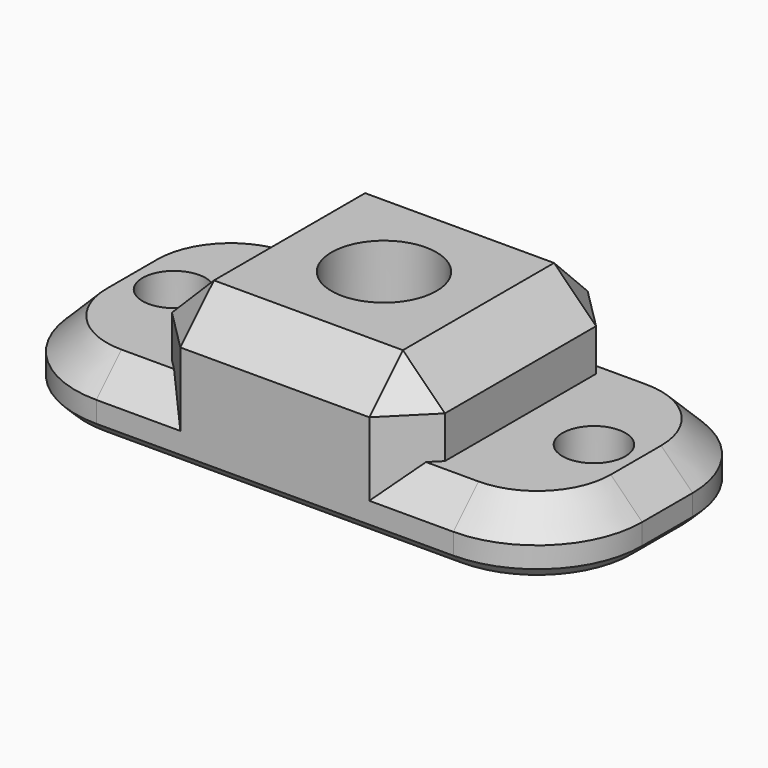
from build123d import *

# Parameters (mm, degrees)
F0_W         = 13
F0_H         = 13
F0_R         = 2.5
F1_DEPTH     = 7
F0_W_2       = 7
F0_R_2       = 1.5
F2_DEPTH     = 3
F3_SIZE      = 2
F4_R         = 5
F5_SIZE      = 1.5
F6_T1_DEPTH  = 3
F6_T3_DEPTH  = 17
F6_T6_ANGLE  = 90
F6_T8_ANGLE  = 90
F6_T10_ANGLE = 90
F6_T12_ANGLE = 90


# Not quite as in the source:
# - a fillet or chamfer that OpenCascade refuses, or shapes differently, is made with other operations: its cross-section is extruded or revolved along the edge and cut away or added


with BuildPart() as f1:
    # F0 (on Top) → F1 (new body)
    with BuildSketch(Plane.XY):
        Rectangle(F0_W, F0_H)
        Circle(F0_R, mode=Mode.SUBTRACT)
    extrude(amount=F1_DEPTH)

    # F0 (on Top) → F2 (join)
    with BuildSketch(Plane.XY):
        with Locations((-10, 0)):
            Rectangle(F0_W_2, F0_H)
        with Locations((-10, 0)):
            Circle(F0_R_2, mode=Mode.SUBTRACT)
        with Locations((10, 0)):
            Rectangle(F0_W_2, F0_H)
        with Locations((10, 0)):
            Circle(F0_R_2, mode=Mode.SUBTRACT)
    extrude(amount=F2_DEPTH)

    # F3
    f3_edges = [f1.edges().sort_by_distance(p)[0] for p in [
        (-2.5, 0, 0),
        (6.5, 0, 7),
        (-6.5, 0, 7),
        (0, -6.5, 7),
        (0, 6.5, 7),
        (-6.5, -6.5, 5),
        (6.5, -6.5, 5),
        (-6.5, 6.5, 5),
        (6.5, 6.5, 5),
    ]]
    chamfer(f3_edges, length=F3_SIZE)

    # F4
    f4_edges = [f1.edges().sort_by_distance(p)[0] for p in [
        (-13.5, 6.5, 1.5),
        (-13.5, -6.5, 1.5),
        (13.5, -6.5, 1.5),
        (13.5, 6.5, 1.5),
    ]]
    fillet(f4_edges, radius=F4_R)

    # F5
    f5_edges = [f1.edges().sort_by_distance(p)[0] for p in [
        (-12.035534, -5.035534, 3),
        (12.035534, -5.035534, 3),
        (7.5, 6.5, 3),
        (12.035534, 5.035534, 3),
        (13.5, 0, 3),
        (7.5, -6.5, 3),
        (-7.5, 6.5, 3),
        (-7.5, -6.5, 3),
        (-13.5, 0, 3),
        (-12.035534, 5.035534, 3),
    ]]
    chamfer(f5_edges, length=F5_SIZE)

    # F6: chamfer of 0.5 on 11 edges, made by hand

    # F6_s2 → F6_t1 (cut)
    with BuildSketch(Plane.XZ.offset(-1.5)):
        Polygon((-13, 0), (-13.5, 0.5), (-13.5, 0), align=None)
        Polygon((13.5, 0.5), (13, 0), (13.5, 0), align=None)
    extrude(amount=F6_T1_DEPTH, mode=Mode.SUBTRACT)

    # F6_s4 → F6_t3 (cut)
    with BuildSketch(Plane.YZ.offset(-8.5)):
        Polygon((6.5, 0.5), (6, 0), (6.5, 0), align=None)
        Polygon((-6.5, 0.5), (-6, 0), (-6.5, 0), align=None)
    extrude(amount=F6_T3_DEPTH, mode=Mode.SUBTRACT)

    # F6_s5 → F6_t6 (revolve, cut)
    with BuildSketch(Plane.YZ.offset(-8.5)):
        Polygon((6, 0), (6.5, 0.5), (6.5, 0), align=None)
    revolve(axis=Axis((-8.5, 1.5, 0), (0, 0, 1)), revolution_arc=F6_T6_ANGLE, mode=Mode.SUBTRACT)

    # F6_s7 → F6_t8 (revolve, cut)
    with BuildSketch(Plane.YZ.offset(-8.5)):
        Polygon((-6, 0), (-6.5, 0.5), (-6.5, 0), align=None)
    revolve(axis=Axis((-8.5, -1.5, 0), (0, 0, -1)), revolution_arc=F6_T8_ANGLE, mode=Mode.SUBTRACT)

    # F6_s9 → F6_t10 (revolve, cut)
    with BuildSketch(Plane.YZ.offset(8.5)):
        Polygon((6.5, 0.5), (6, 0), (6.5, 0), align=None)
    revolve(axis=Axis((8.5, 1.5, 0), (0, 0, -1)), revolution_arc=F6_T10_ANGLE, mode=Mode.SUBTRACT)

    # F6_s11 → F6_t12 (revolve, cut)
    with BuildSketch(Plane.YZ.offset(8.5)):
        Polygon((-6.5, 0.5), (-6, 0), (-6.5, 0), align=None)
    revolve(axis=Axis((8.5, -1.5, 0), (0, 0, 1)), revolution_arc=F6_T12_ANGLE, mode=Mode.SUBTRACT)

    # F6_s13 → F6_t14 (revolve, cut)
    with BuildSketch(Plane.XZ):
        Polygon((4.7071067812, 0), (4.3535533906, 0.1464466094), (4.5, 0), align=None)
    revolve(axis=Axis((0, 0, 0), (0, 0, 1)), mode=Mode.SUBTRACT)

    # F6_s15 → F6_t16 (revolve, cut)
    with BuildSketch(Plane.XZ):
        Polygon((11.5, 0.5), (12, 0), (11.5, 0), align=None)
    revolve(axis=Axis((10, 0, 0), (0, 0, 1)), mode=Mode.SUBTRACT)

    # F6_s17 → F6_t18 (revolve, cut)
    with BuildSketch(Plane.XZ):
        Polygon((-8, 0), (-8.5, 0.5), (-8.5, 0), align=None)
    revolve(axis=Axis((-10, 0, 0), (0, 0, 1)), mode=Mode.SUBTRACT)


solid = f1.part
